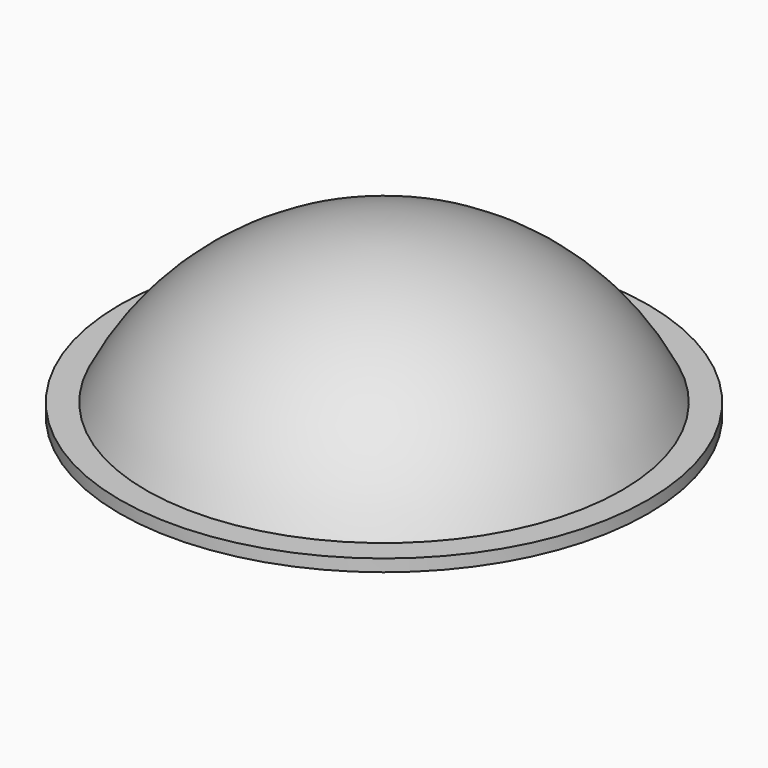
from build123d import *


# Not quite as in the source:
# - a feature of the source that left no trace in its solid (it failed there, or was rolled back) is left out


with BuildPart() as f1:
    # F0 (on Front) → F1 (revolve)
    with BuildSketch(Plane.XZ):
        with BuildLine():
            ThreePointArc((0, 12), (11.1238371214, 8.7427789702), (18.7339, 0))
            Line((18.7339, 0), (21.7339, 0))
            Line((21.7339, 0), (21.7339, 1))
            Line((21.7339, 1), (19.7339, 1))
            Line((19.7339, 1), (19.5869427433, 1))
            ThreePointArc((19.5869427433, 1), (11.5378542852, 9.9005842829), (0, 13.2))
            Line((0, 13.2), (0, 12))
        make_face()
    revolve(axis=Axis((0, 0, 12.6), (0, 0, -1)))


solid = f1.part
